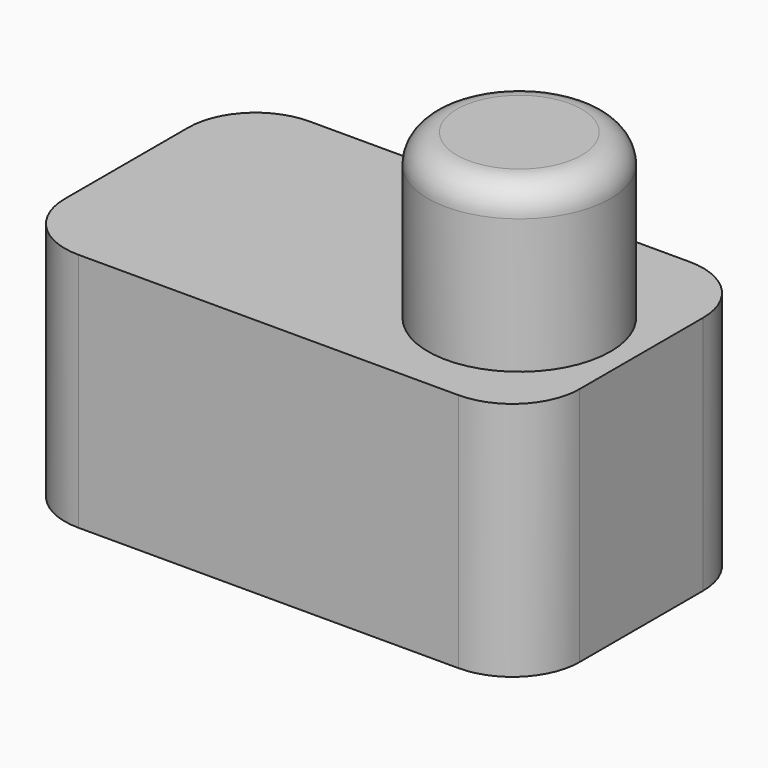
from build123d import *

# Parameters (mm, degrees)
F0_W      = 53.5574629903
F0_H      = 30.0444331951
F1_DEPTH  = 25
F2_R      = 9.492451093
F3_DEPTH  = 17
F4_R      = 3
F5_R      = 7
F6_R      = 7
F7_R      = 7
F8_R      = 7
F11_W     = 10.4502402246
F11_H     = 5.4117300315
F12_DEPTH = 2


# Not quite as in the source:
# - the program builds the solid bodies; features that only make, move or delete a surface that nothing else refers to are left out


with BuildPart() as f1:
    # F0 (on Top) → F1 (new body)
    with BuildSketch(Plane.XY):
        with Locations((-33.1235192716, 21.5536148753)):
            Rectangle(F0_W, F0_H)
    extrude(amount=F1_DEPTH)

    # F2 (on face) → F3 (join)
    with BuildSketch(Plane.XY.offset(25)):
        with Locations((-17.996661365, 20.2366635203)):
            Circle(F2_R)
    extrude(amount=F3_DEPTH)

    # F4
    f4_edges = [f1.edges().sort_by_distance(p)[0] for p in [
        (-27.489112, 20.236664, 42),
    ]]
    fillet(f4_edges, radius=F4_R)

    # F5
    f5_edges = [f1.edges().sort_by_distance(p)[0] for p in [
        (-6.344788, 36.575831, 12.5),
    ]]
    fillet(f5_edges, radius=F5_R)

    # F6
    f6_edges = [f1.edges().sort_by_distance(p)[0] for p in [
        (-59.902251, 36.575831, 12.5),
    ]]
    fillet(f6_edges, radius=F6_R)

    # F7
    f7_edges = [f1.edges().sort_by_distance(p)[0] for p in [
        (-59.902251, 6.531398, 12.5),
    ]]
    fillet(f7_edges, radius=F7_R)

    # F8
    f8_edges = [f1.edges().sort_by_distance(p)[0] for p in [
        (-6.344788, 6.531398, 12.5),
    ]]
    fillet(f8_edges, radius=F8_R)

    # F11 (on face) → F12 (join)
    with BuildSketch(Plane(origin=(0, 36.5758314729, 0), x_dir=(-1, 0, 0), z_dir=(0, 1, 0))):
        with Locations((43.4804502875, 4.3853675597)):
            Rectangle(F11_W, F11_H)
    extrude(amount=F12_DEPTH)


solid = f1.part
